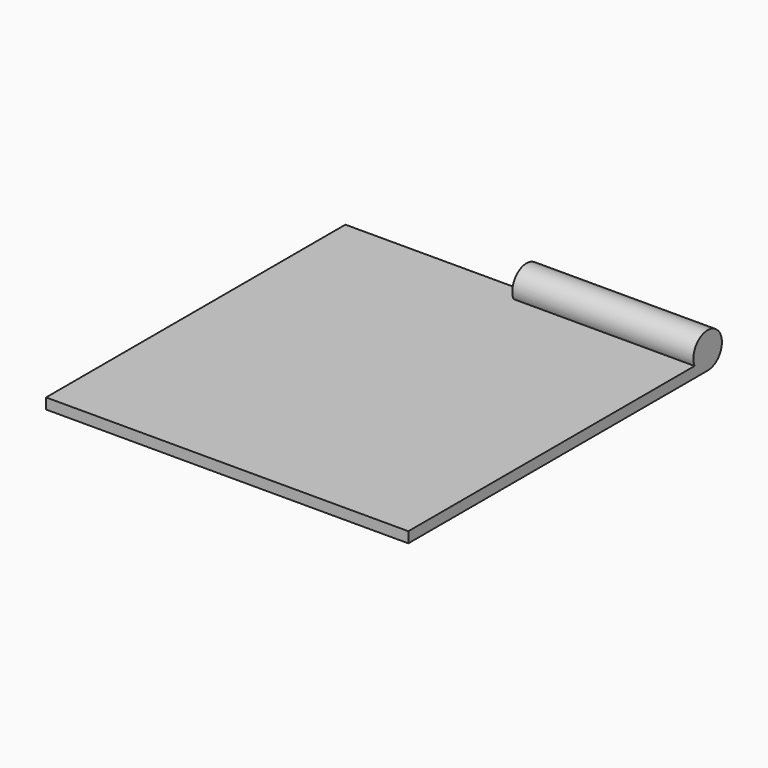
from build123d import *

# Parameters (mm, degrees)
F0_W     = 61
F0_H     = 63
F1_DEPTH = 1.8
F3_DEPTH = 30.5


with BuildPart() as f1:
    # F0 (on Top) → F1 (new body)
    with BuildSketch(Plane.XY):
        with Locations((30.5, -31.5)):
            Rectangle(F0_W, F0_H)
    extrude(amount=F1_DEPTH)

    # F2 (on face) → F3 (join)
    with BuildSketch(Plane.YZ.offset(61)):
        with BuildLine():
            Line((0, 1.8), (0, 0))
            ThreePointArc((0, 0), (2.1213203436, 0.8786796564), (3, 3))
            ThreePointArc((3, 3), (-0.6129289311, 5.9367189388), (-2.749545417, 1.8))
            Line((-2.749545417, 1.8), (0, 1.8))
        make_face()
        with BuildLine():
            ThreePointArc((-2.749545417, 1.8), (-1.6431676725, 0.4900199204), (0, 0))
            Line((0, 0), (0, 1.8))
            Line((0, 1.8), (-2.749545417, 1.8))
        make_face()
    extrude(amount=-F3_DEPTH)


solid = f1.part
